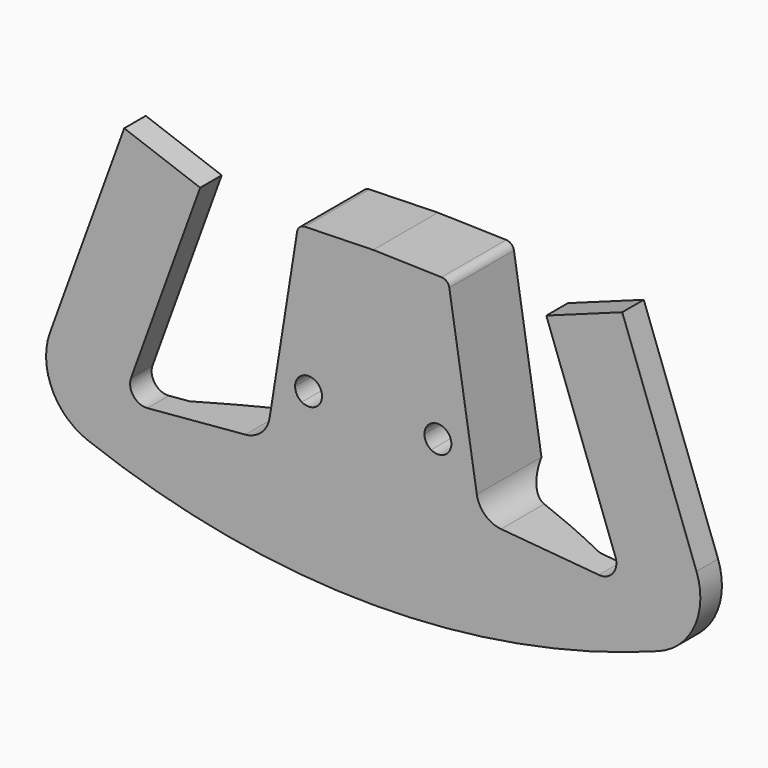
from build123d import *

# Parameters (mm, degrees)
F0_W        = 46
F0_H        = 30
F0_R        = 2.5
F0_R_2      = 1.25
F1_DEPTH    = 10
F2_DEPTH    = 20
F3_R        = 2.5
F4_DEPTH    = 30
F5_DEPTH    = 20
F6_DEPTH    = 16
F7_DEPTH    = 5
F8_T4_ANGLE = 69.3687445925
F9_W        = 6
F9_H        = 8
F10_REACH   = 90.001


# Not quite as in the source:
# - a fillet or chamfer that OpenCascade refuses, or shapes differently, is made with other operations: its cross-section is extruded or revolved along the edge and cut away or added
# - a feature names something its author has since deleted; it is built from what else it names


with BuildPart() as f1:
    # F0 (on Front) → F1 (new body)
    with BuildSketch(Plane.XZ):
        with BuildLine():
            Line((25.3649208898, 103.335796171), (0, 104))
            Line((0, 104), (-25.3649208898, 103.335796171))
            ThreePointArc((-25.3649208898, 103.335796171), (-27.2638102508, 102.5928847735), (-28.2491977972, 100.8077490551))
            Line((-28.2491977972, 100.8077490551), (-38.4537664635, 36.6060519686))
            ThreePointArc((-38.4537664635, 36.6060519686), (-41.511810122, 30.8603986419), (-47.4582348771, 28.2138545179))
            Line((-47.4582348771, 28.2138545179), (-83.8130942566, 25.0332164582))
            ThreePointArc((-83.8130942566, 25.0332164582), (0, 9.922889923), (83.8130942566, 25.0332164582))
            Line((83.8130942566, 25.0332164582), (47.4582348771, 28.2138545179))
            ThreePointArc((47.4582348771, 28.2138545179), (41.511810122, 30.8603986419), (38.4537664635, 36.6060519686))
            Line((38.4537664635, 36.6060519686), (28.2491977972, 100.8077490551))
            ThreePointArc((28.2491977972, 100.8077490551), (27.2638102508, 102.5928847735), (25.3649208898, 103.335796171))
        make_face()
        with Locations((0, 83)):
            Rectangle(F0_W, F0_H, mode=Mode.SUBTRACT)
        with Locations((0, 83)):
            Rectangle(F0_W, F0_H)
        with Locations((-17, 75)):
            Circle(F0_R, mode=Mode.SUBTRACT)
        with Locations((-17, 93)):
            Circle(F0_R, mode=Mode.SUBTRACT)
        with Locations((17, 75)):
            Circle(F0_R, mode=Mode.SUBTRACT)
        with Locations((17, 93)):
            Circle(F0_R, mode=Mode.SUBTRACT)
        with Locations((17, 93)):
            Circle(F0_R)
        with Locations((17, 93)):
            Circle(F0_R_2, mode=Mode.SUBTRACT)
        with Locations((17, 75)):
            Circle(F0_R)
        with Locations((17, 75)):
            Circle(F0_R_2, mode=Mode.SUBTRACT)
        with Locations((-17, 93)):
            Circle(F0_R)
        with Locations((-17, 93)):
            Circle(F0_R_2, mode=Mode.SUBTRACT)
        with Locations((-17, 75)):
            Circle(F0_R)
        with Locations((-17, 75)):
            Circle(F0_R_2, mode=Mode.SUBTRACT)
        with Locations((17, 93)):
            Circle(F0_R_2)
        with Locations((-17, 93)):
            Circle(F0_R_2)
        with Locations((-17, 75)):
            Circle(F0_R_2)
        with Locations((17, 75)):
            Circle(F0_R_2)
        with BuildLine():
            ThreePointArc((83.8130942566, 25.0332164582), (0, 9.922889923), (-83.8130942566, 25.0332164582))
            ThreePointArc((-83.8130942566, 25.0332164582), (-89.0331441362, 27.330093377), (-89.9007085466, 32.9667498611))
            Line((-89.9007085466, 32.9667498611), (-64.2491977972, 103.44369642))
            Line((-64.2491977972, 103.44369642), (-92.4399764208, 113.7043007198))
            Line((-92.4399764208, 113.7043007198), (-120, 37.9837582563))
            ThreePointArc((-120, 37.9837582563), (-119.2581515912, 19.7607795149), (-105.9210620665, 7.3209508875))
            ThreePointArc((-105.9210620665, 7.3209508875), (-53.8344000907, -7.1302379745), (0, -12))
            ThreePointArc((0, -12), (53.8344000907, -7.1302379745), (105.9210620665, 7.3209508875))
            ThreePointArc((105.9210620665, 7.3209508875), (119.2581515912, 19.7607795149), (120, 37.9837582563))
            Line((120, 37.9837582563), (92.4399764208, 113.7043007198))
            Line((92.4399764208, 113.7043007198), (64.2491977972, 103.44369642))
            Line((64.2491977972, 103.44369642), (89.9007085466, 32.9667498611))
            ThreePointArc((89.9007085466, 32.9667498611), (89.0331441362, 27.330093377), (83.8130942566, 25.0332164582))
        make_face()
    extrude(amount=F1_DEPTH)

    # F0 (on Front) → F2 (join)
    with BuildSketch(Plane.XZ):
        with BuildLine():
            Line((25.3649208898, 103.335796171), (0, 104))
            Line((0, 104), (-25.3649208898, 103.335796171))
            ThreePointArc((-25.3649208898, 103.335796171), (-27.2638102508, 102.5928847735), (-28.2491977972, 100.8077490551))
            Line((-28.2491977972, 100.8077490551), (-38.4537664635, 36.6060519686))
            ThreePointArc((-38.4537664635, 36.6060519686), (-41.511810122, 30.8603986419), (-47.4582348771, 28.2138545179))
            Line((-47.4582348771, 28.2138545179), (-83.8130942566, 25.0332164582))
            ThreePointArc((-83.8130942566, 25.0332164582), (0, 9.922889923), (83.8130942566, 25.0332164582))
            Line((83.8130942566, 25.0332164582), (47.4582348771, 28.2138545179))
            ThreePointArc((47.4582348771, 28.2138545179), (41.511810122, 30.8603986419), (38.4537664635, 36.6060519686))
            Line((38.4537664635, 36.6060519686), (28.2491977972, 100.8077490551))
            ThreePointArc((28.2491977972, 100.8077490551), (27.2638102508, 102.5928847735), (25.3649208898, 103.335796171))
        make_face()
        with Locations((0, 83)):
            Rectangle(F0_W, F0_H, mode=Mode.SUBTRACT)
    extrude(amount=-F2_DEPTH)

    # F3 (on face) → F4 (cut, through all)
    with BuildSketch(Plane.XZ.offset(10)):
        with Locations((-24, 50)):
            Circle(F3_R)
        with Locations((24, 50)):
            Circle(F3_R)
    extrude(amount=-F4_DEPTH, mode=Mode.SUBTRACT)

    # F3 (on face) → F5 (cut, through all)
    with BuildSketch(Plane.XZ.offset(10)):
        Polygon((-21.5, 45.6698729811), (-19, 50), (-21.5, 54.3301270189), (-26.5, 54.3301270189), (-29, 50), (-26.5, 45.6698729811), align=None)
        with Locations((-24, 50)):
            Circle(F3_R, mode=Mode.SUBTRACT)
        Polygon((26.5, 45.6698729811), (29, 50), (26.5, 54.3301270189), (21.5, 54.3301270189), (19, 50), (21.5, 45.6698729811), align=None)
        with Locations((24, 50)):
            Circle(F3_R, mode=Mode.SUBTRACT)
    extrude(amount=-F5_DEPTH, mode=Mode.SUBTRACT)

    # F3 (on face) → F6 (cut, through all)
    with BuildSketch(Plane.XZ.offset(10)):
        with BuildLine():
            ThreePointArc((-29, 50), (-28.3301270189, 47.5), (-26.5, 45.6698729811))
            Line((-26.5, 45.6698729811), (-29, 50))
        make_face()
        with BuildLine():
            Line((-29, 50), (-26.5, 54.3301270189))
            ThreePointArc((-26.5, 54.3301270189), (-28.3301270189, 52.5), (-29, 50))
        make_face()
        with BuildLine():
            Line((-26.5, 54.3301270189), (-21.5, 54.3301270189))
            ThreePointArc((-21.5, 54.3301270189), (-24, 55), (-26.5, 54.3301270189))
        make_face()
        with BuildLine():
            Line((-21.5, 54.3301270189), (-19, 50))
            ThreePointArc((-19, 50), (-19.6698729811, 52.5), (-21.5, 54.3301270189))
        make_face()
        with BuildLine():
            ThreePointArc((-21.5, 45.6698729811), (-19.6698729811, 47.5), (-19, 50))
            Line((-19, 50), (-21.5, 45.6698729811))
        make_face()
        with BuildLine():
            ThreePointArc((-26.5, 45.6698729811), (-24, 45), (-21.5, 45.6698729811))
            Line((-21.5, 45.6698729811), (-26.5, 45.6698729811))
        make_face()
        with BuildLine():
            Line((19, 50), (21.5, 54.3301270189))
            ThreePointArc((21.5, 54.3301270189), (19.6698729811, 52.5), (19, 50))
        make_face()
        with BuildLine():
            Line((21.5, 54.3301270189), (26.5, 54.3301270189))
            ThreePointArc((26.5, 54.3301270189), (24, 55), (21.5, 54.3301270189))
        make_face()
        with BuildLine():
            Line((26.5, 54.3301270189), (29, 50))
            ThreePointArc((29, 50), (28.3301270189, 52.5), (26.5, 54.3301270189))
        make_face()
        with BuildLine():
            ThreePointArc((26.5, 45.6698729811), (28.3301270189, 47.5), (29, 50))
            Line((29, 50), (26.5, 45.6698729811))
        make_face()
        with BuildLine():
            ThreePointArc((21.5, 45.6698729811), (24, 45), (26.5, 45.6698729811))
            Line((26.5, 45.6698729811), (21.5, 45.6698729811))
        make_face()
        with BuildLine():
            ThreePointArc((19, 50), (19.6698729811, 47.5), (21.5, 45.6698729811))
            Line((21.5, 45.6698729811), (19, 50))
        make_face()
    extrude(amount=-F6_DEPTH, mode=Mode.SUBTRACT)

    # F0 (on Front) → F7 (join)
    with BuildSketch(Plane.XZ):
        with Locations((17, 93)):
            Circle(F0_R)
        with Locations((17, 93)):
            Circle(F0_R_2, mode=Mode.SUBTRACT)
        with Locations((17, 75)):
            Circle(F0_R)
        with Locations((17, 75)):
            Circle(F0_R_2, mode=Mode.SUBTRACT)
        with Locations((-17, 75)):
            Circle(F0_R)
        with Locations((-17, 75)):
            Circle(F0_R_2, mode=Mode.SUBTRACT)
        with Locations((-17, 93)):
            Circle(F0_R)
        with Locations((-17, 93)):
            Circle(F0_R_2, mode=Mode.SUBTRACT)
    extrude(amount=-F7_DEPTH)

    # F8: chamfer of 23.2 on 1 edges, made by hand


with BuildPart() as f8_tool2:
    # F8_s3 → F8_t4 (revolve)
    with BuildSketch(Plane(origin=(-116.9473505208, 0, 80.9310017088), x_dir=(0, 1, 0), z_dir=(-0.8222992842, 0, 0.5690552585))):
        Polygon((20, 11.2885865066), (-3.2, 34.4885865066), (20, 34.4885865066), align=None)
    revolve(axis=Axis((0, 20, 249.922889923), (0, -1, 0)), revolution_arc=F8_T4_ANGLE)

    split(bisect_by=Plane.XZ, keep=Keep.BOTTOM)


with BuildPart() as f1_1:
    add(f1.part)

    # F8_t1: cut F8_tool2
    add(f8_tool2.part, mode=Mode.SUBTRACT)

    f10_end = f1_1.faces().sort_by_distance((0, 10, 23.1228899231))[0]
    # F9 (on face) → F10 (cut, up to a face of the model that its end follows)
    with BuildSketch(Plane.XY.offset(68)):
        with Locations((10, 8)):
            Rectangle(F9_W, F9_H)
        with Locations((-10, 8)):
            Rectangle(F9_W, F9_H)
    f10_long = extrude(amount=-F10_REACH, mode=Mode.PRIVATE)
    add(split(f10_long, bisect_by=f10_end, keep=Keep.BOTTOM, mode=Mode.PRIVATE), mode=Mode.SUBTRACT)


solid = f1_1.part
